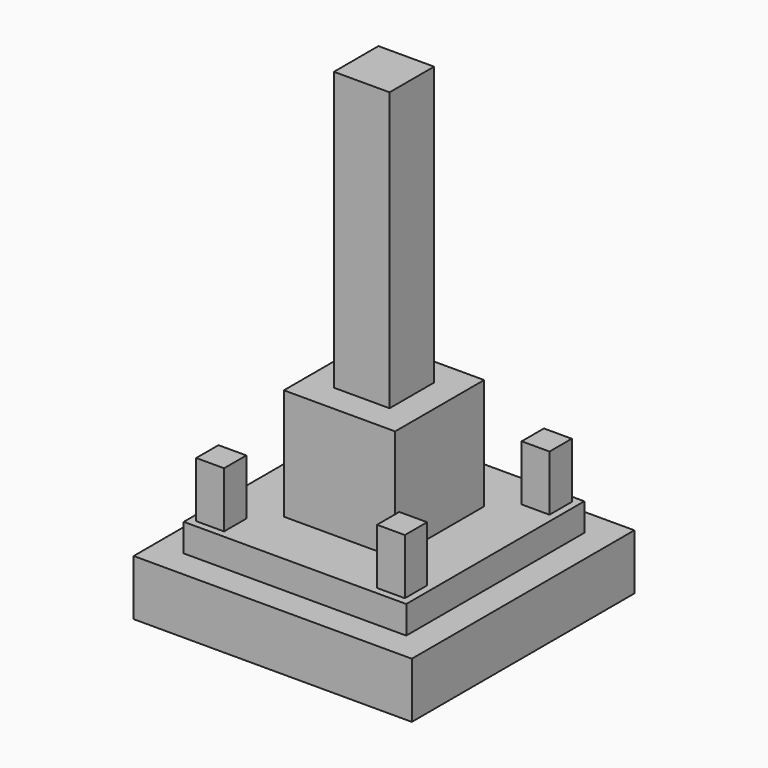
from build123d import *

# Parameters (mm, degrees)
F0_W      = 25.4
F0_H      = 25.4
F1_DEPTH  = 5.08
F2_W      = 20.32
F2_H      = 20.32
F3_DEPTH  = 2.54
F4_W      = 10.16
F4_H      = 10.16
F5_DEPTH  = 10.16
F6_W      = 5.08
F6_H      = 5.08
F7_DEPTH  = 25.4
F8_W      = 2.54
F8_H      = 2.54
F9_DEPTH  = 5.08
F10_R     = 0.635
F11_DEPTH = 0.254
F13_R     = 2.2046300475
F14_DEPTH = 25.4


# Not quite as in the source:
# - a fillet or chamfer that OpenCascade refuses, or shapes differently, is made with other operations: its cross-section is extruded or revolved along the edge and cut away or added


with BuildPart() as f1:
    # F0 (on Top) → F1 (new body)
    with BuildSketch(Plane.XY):
        with Locations((12.7, -12.7)):
            Rectangle(F0_W, F0_H)
    extrude(amount=F1_DEPTH)

    # F2 (on face) → F3 (join)
    with BuildSketch(Plane.XY.offset(5.08)):
        with Locations((12.7, -12.7)):
            Rectangle(F2_W, F2_H)
    extrude(amount=F3_DEPTH)

    # F4 (on face) → F5 (join)
    with BuildSketch(Plane.XY.offset(7.62)):
        with Locations((12.7, -12.7)):
            Rectangle(F4_W, F4_H)
    extrude(amount=F5_DEPTH)

    # F6 (on face) → F7 (join)
    with BuildSketch(Plane.XY.offset(17.78)):
        with Locations((12.7, -12.7)):
            Rectangle(F6_W, F6_H)
    extrude(amount=F7_DEPTH)

    # F8 (on face) → F9 (join)
    with BuildSketch(Plane.XY.offset(7.62)):
        with Locations((4.445, -4.445)):
            Rectangle(F8_W, F8_H)
        with Locations((20.955, -4.445)):
            Rectangle(F8_W, F8_H)
        with Locations((20.955, -20.955)):
            Rectangle(F8_W, F8_H)
        with Locations((4.445, -20.955)):
            Rectangle(F8_W, F8_H)
    extrude(amount=F9_DEPTH)

    # F10 (on face) → F11 (join)
    with BuildSketch(Plane.XZ.offset(22.225)):
        with Locations((4.445, 11.43)):
            Circle(F10_R)
    extrude(amount=F11_DEPTH)

    # F12: fillet of radius 0.8636 on 1 edges, made by hand


with BuildPart() as f12_tool2:
    # F12_s3 → F12_t4 (revolve)
    with BuildSketch(Plane.XY.offset(11.43)):
        with BuildLine():
            ThreePointArc((5.08, -21.6154), (4.9031400964, -22.1390344145), (4.445, -22.4481946926))
            Line((4.445, -22.4481946926), (4.445, -22.479))
            Line((4.445, -22.479), (5.08, -22.479))
            Line((5.08, -22.479), (5.08, -21.6154))
        make_face()
    revolve(axis=Axis((4.445, -22.479, 11.43), (0, -1, 0)))

    split(bisect_by=Plane.XZ.offset(22.225), keep=Keep.TOP)


with BuildPart() as f1_1:
    add(f1.part)

    # F12_t1: cut F12_tool2
    add(f12_tool2.part, mode=Mode.SUBTRACT)

    # F13 (on face) → F14 (cut)
    with BuildSketch(Plane.XZ.offset(22.225)):
        with Locations((4.445, 11.43)):
            Circle(F13_R)
    extrude(amount=F14_DEPTH, mode=Mode.SUBTRACT)


solid = f1_1.part
